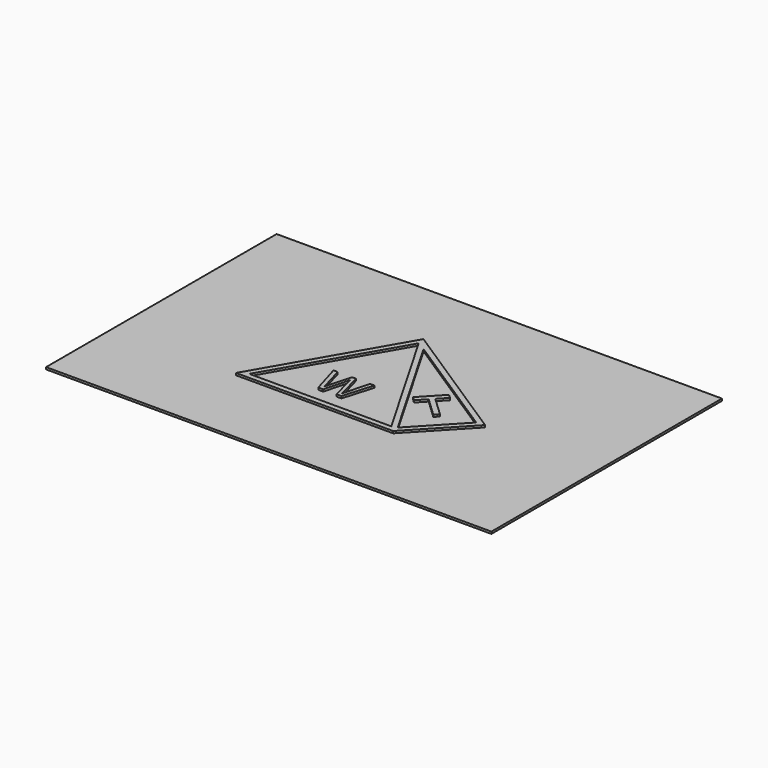
from build123d import *

# Parameters (mm, degrees)
F0_W         = 85
F0_H         = 55
F1_DEPTH     = 0.4
F3_DEPTH     = 0.4
F4_TEXT_SIZE = 8.3333333333
F5_DEPTH     = 0.4


# Not quite as in the source:
# - Text() gives the source's letters only with a copy of the font that has no kerning and outlines rounded to 1/6400 em; it was checked with that copy


with BuildPart() as f1:
    # F0 (on Top) → F1 (new body)
    with BuildSketch(Plane.XY):
        Rectangle(F0_W, F0_H)
    extrude(amount=F1_DEPTH)

    # F2 (on face) → F3 (join)
    with BuildSketch(Plane.XY.offset(0.4)):
        Polygon((20.7652670797, -1.8392873462), (-3.7396327031, 14.0902642101), (-18.7396327031, -11.8904979035), (11.2603672969, -11.8904979035), align=None)
        Polygon((6.3882751176, -10.8904979035), (-17.0075818955, -10.8904979035), (-6.5965332599, 7.1419672935), (-3.4509575685, 12.5902642101), (10.1056667585, -10.8904979035), align=None, mode=Mode.SUBTRACT)
        Polygon((-1.7130832558, 11.5801776034), (19.2144094908, -2.0238598588), (11.0971054812, -10.6077201437), align=None, mode=Mode.SUBTRACT)
    extrude(amount=F3_DEPTH)

    # F4 (on face) → F5 (join)
    with BuildSketch(Plane.XY.offset(0.4)):
        Polygon((12.6254242083, -4.0203356419), (12.9689668658, -3.6570472681), (13.3125095232, -3.2937588943), (9.6796257853, 0.1416676799), (11.1987832394, 1.7481413713), (10.4722064918, 2.4352266862), (8.6095063803, 0.4654646209), (6.7468062687, -1.5042974443), (7.4733830163, -2.1913827592), (8.9925404704, -0.5849090677), align=None)
        with Locations((-7.9473149947, -7.9001168467)):
            Text('W', F4_TEXT_SIZE, font='Arimo', text_align=(TextAlign.LEFT, TextAlign.BOTTOM))
    extrude(amount=F5_DEPTH)


solid = f1.part
